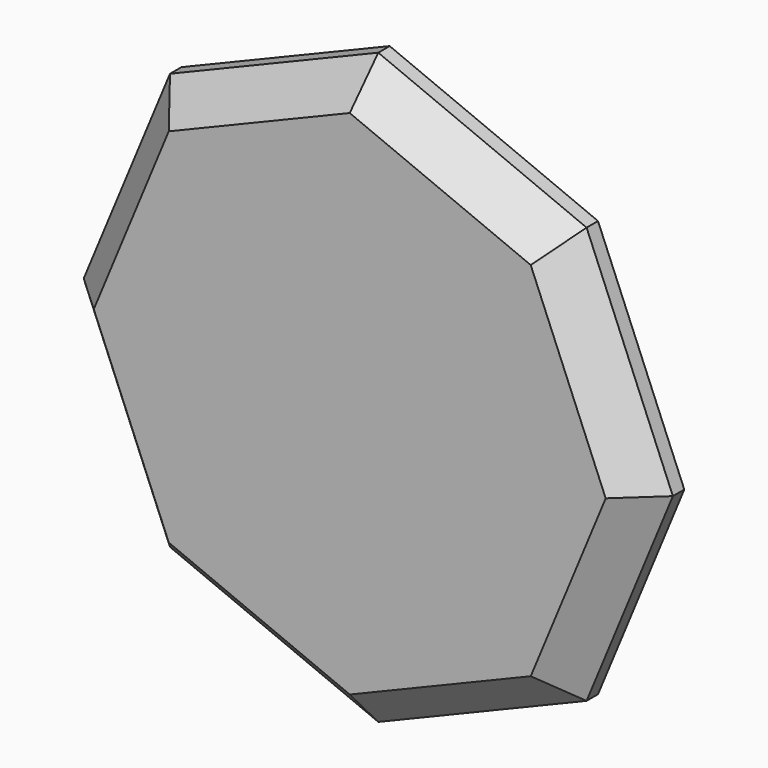
from build123d import *

# Parameters (mm, degrees)
F1_DEPTH = 50
F2_SIZE  = 49.99999
F3_DEPTH = 20


# Not quite as in the source:
# - a fillet or chamfer is up to 0.001 mm smaller than in the source, because OpenCascade refuses the exact size


with BuildPart() as f1:
    # F0 (on Front) → F1 (new body)
    with BuildSketch(Plane.XZ):
        Polygon((291.8585808619, -291.8585808619), (412.7503633499, 0), (291.8585808619, 291.8585808619), (0, 412.7503633499), (-291.8585808619, 291.8585808619), (-412.7503633499, 0), (-291.8585808619, -291.8585808619), (0, -412.7503633499), align=None)
    extrude(amount=F1_DEPTH)

    # F2 (size 50 in the source; OpenCascade refuses exactly that, so slightly less here)
    f2_edges = [f1.edges().sort_by_distance(p)[0] for p in [
        (-352.304472, -50, -145.92929),
        (-145.92929, -50, -352.304472),
        (145.92929, -50, -352.304472),
        (352.304472, -50, -145.92929),
        (352.304472, -50, 145.92929),
        (145.92929, -50, 352.304472),
        (-145.92929, -50, 352.304472),
        (-352.304472, -50, 145.92929),
    ]]
    chamfer(f2_edges, length=F2_SIZE)

    # F0 (on Front) → F3 (join)
    with BuildSketch(Plane.XZ):
        Polygon((291.8585808619, -291.8585808619), (412.7503633499, 0), (291.8585808619, 291.8585808619), (0, 412.7503633499), (-291.8585808619, 291.8585808619), (-412.7503633499, 0), (-291.8585808619, -291.8585808619), (0, -412.7503633499), align=None)
    extrude(amount=-F3_DEPTH)


solid = f1.part
